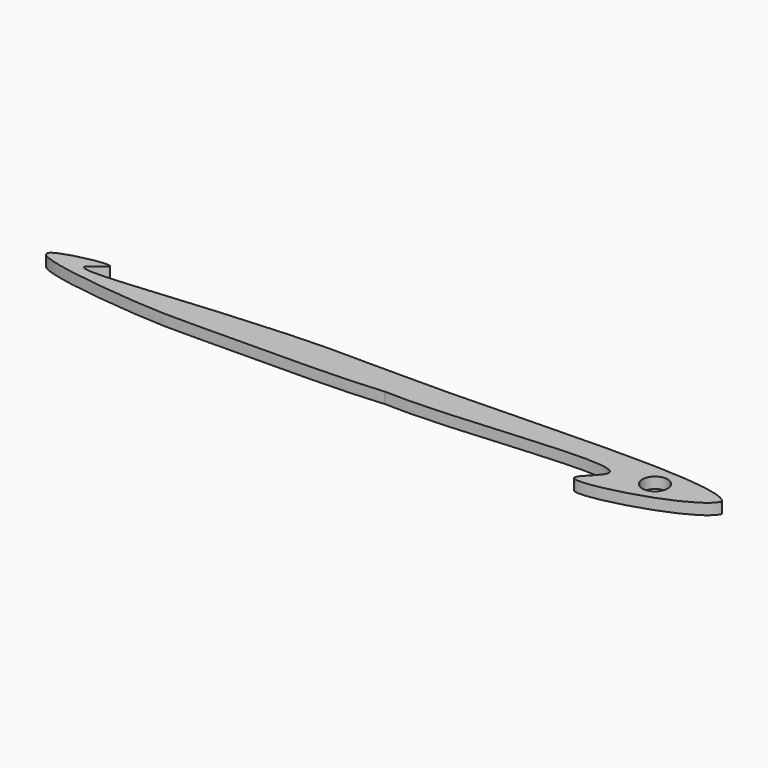
from build123d import *

# Parameters (mm, degrees)
F1_DEPTH = 1
F2_R     = 1.1487741976
F3_DEPTH = 25


with BuildPart() as f1:
    # F0 (on Top) → F1 (new body)
    with BuildSketch(Plane.XY):
        with BuildLine():
            add(Edge.make_bspline(
                [(0, 0.9594753346), (8.6504682046, 0.8386531946), (27.9755286493, 2.3259491006), (29.3201971907, 0)],
                knots=[0.372422483, 0.372422483, 0.372422483, 0.372422483, 1, 1, 1, 1], degree=3))
            add(Edge.make_bspline(
                [(0, 0.9594753346), (-3.0588429709, 0.9110639463), (-4.9191047941, 1.0010118294), (-7.2686058101, 0.9751205946)],
                knots=[0, 0, 0, 0, 0.1136801708, 0.1136801708, 0.1136801708, 0.1136801708], degree=3))
            add(Edge.make_bspline(
                [(-10.2862044503, 0), (-9.109134082, 0.5199849001), (-8.1653764752, 0.8160683552), (-7.2686058101, 0.9751205946)],
                knots=[0, 0, 0, 0, 0.1160171443, 0.1160171443, 0.1160171443, 0.1160171443], degree=3))
            add(Edge.make_bspline(
                [(-10.2862044503, 0), (-6.5077329836, 0), (-4.9312894429, -1.5310231402), (0, -1.7503085824)],
                knots=[0, 0, 0, 0, 0.2546522806, 0.2546522806, 0.2546522806, 0.2546522806], degree=3))
            add(Edge.make_bspline(
                [(0, -1.7503085824), (6.8740786765, -2.0559863163), (25.0676874581, 0.9913012801), (15.008036825, -5.6959945314), (28.3728268523, -2.1476281598), (29.3201971907, 0)],
                knots=[0.2546522806, 0.2546522806, 0.2546522806, 0.2546522806, 0.6096303918, 0.7368667067, 1, 1, 1, 1], degree=3))
        make_face()
        with BuildLine():
            add(Edge.make_bspline(
                [(-10.2862044503, 0), (-9.109134082, 0.5199849001), (-8.1653764752, 0.8160683552), (-7.2686058101, 0.9751205946)],
                knots=[0, 0, 0, 0, 0.1160171443, 0.1160171443, 0.1160171443, 0.1160171443], degree=3))
            add(Edge.make_bspline(
                [(-7.2686058101, 0.9751205946), (-7.5624213285, 0.9718827809), (-11.4169906772, 0.9073211469), (-20.6149830719, 0.1871349563), (-30.8962958204, -0.8400259059), (-25.2382537195, 1.9638712633), (-37.1883742413, -0.4259963698), (-21.2865303674, -2.2825934057), (-17.3997042774, -2.1240190962), (-3.795313327, -2.1409456687), (0, -1.7503085824)],
                knots=[0.1136801708, 0.1136801708, 0.1136801708, 0.1136801708, 0.1278963801, 0.2954494802, 0.4098552425, 0.468789908, 0.5670047062, 0.7030570953, 0.8194052271, 1, 1, 1, 1], degree=3))
            add(Edge.make_bspline(
                [(-10.2862044503, 0), (-6.5077329836, 0), (-4.9312894429, -1.5310231402), (0, -1.7503085824)],
                knots=[0, 0, 0, 0, 0.2546522806, 0.2546522806, 0.2546522806, 0.2546522806], degree=3))
        make_face()
    extrude(amount=F1_DEPTH)

    # F2 (on face) → F3 (cut)
    with BuildSketch(Plane.XY.offset(1)):
        with Locations((23.9077936858, -0.8492149063)):
            Circle(F2_R)
    extrude(amount=-F3_DEPTH, mode=Mode.SUBTRACT)


solid = f1.part
